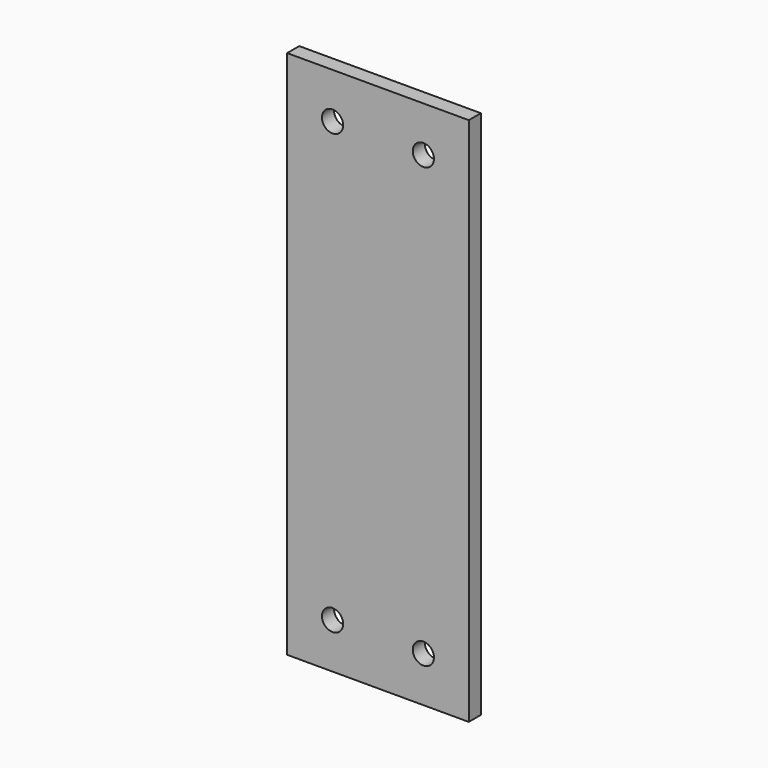
from build123d import *

# Parameters (mm, degrees)
F0_W     = 120
F0_H     = 350
F0_R     = 7
F1_DEPTH = 10


# Not quite as in the source:
# - a feature names something its author has since deleted; it is built from what else it names


with BuildPart() as f1:
    # F0 (on Front) → F1 (new body)
    with BuildSketch(Plane.XZ):
        Rectangle(F0_W, F0_H)
        with Locations((-30, -145)):
            Circle(F0_R, mode=Mode.SUBTRACT)
        with Locations((30, -145)):
            Circle(F0_R, mode=Mode.SUBTRACT)
        with Locations((-30, 145)):
            Circle(F0_R, mode=Mode.SUBTRACT)
        with Locations((30, 145)):
            Circle(F0_R, mode=Mode.SUBTRACT)
    extrude(amount=F1_DEPTH)


solid = f1.part
